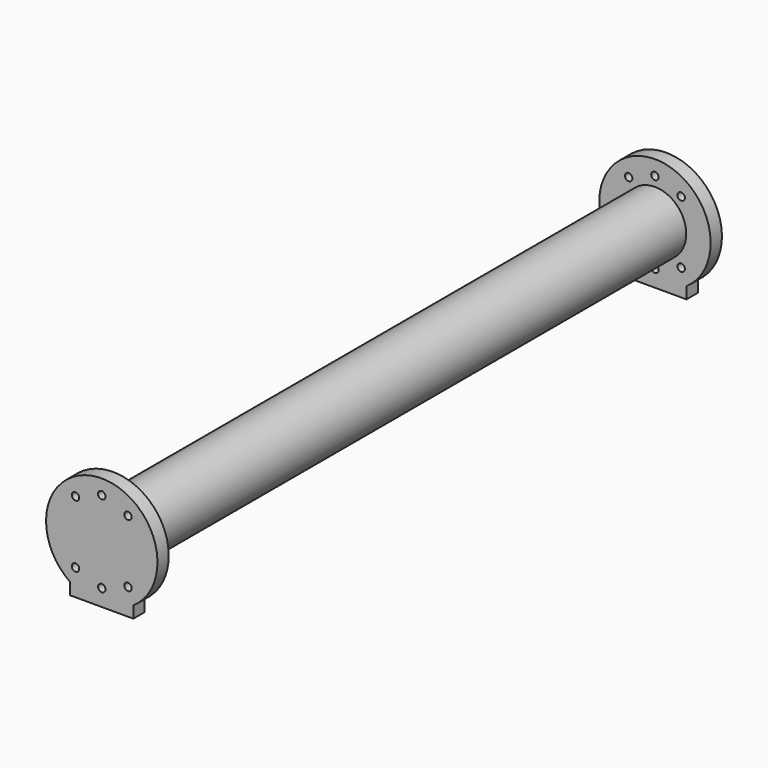
from build123d import *

# Parameters (mm, degrees)
F0_R      = 84.2
F0_R_2    = 76.2
F1_DEPTH  = 912
F2_R      = 75
F3_DEPTH  = 10
F4_R      = 10
F5_DEPTH  = 10
F8_DEPTH  = 38
F9_R      = 10
F10_DEPTH = 38


# Not quite as in the source:
# - a pattern or mirror of a feature is missing from the dataset's text; its kind, count and spacing are read off the source's solid
# - a feature names something its author has since deleted; it is built from what else it names


with BuildPart() as f1:
    # F0 (on Front) → F1 (new body, symmetric)
    with BuildSketch(Plane.XZ):
        Circle(F0_R)
        Circle(F0_R_2, mode=Mode.SUBTRACT)
    extrude(amount=F1_DEPTH, both=True)

    # F7 (on face) → F8 (join)
    with BuildSketch(Plane.XZ.offset(912)):
        with BuildLine():
            Line((85, -155), (85, -123.5920709431))
            ThreePointArc((85, -123.5920709431), (0, 150), (-85, -123.5920709431))
            Line((-85, -123.5920709431), (-85, -155))
            Line((-85, -155), (85, -155))
        make_face()
    f8 = extrude(amount=F8_DEPTH)

    # F8_copies: F8 across plane
    add(f8.mirror(Plane.ZX))

    # F9 (on face) → F10 (cut, through all)
    with BuildSketch(Plane.XZ.offset(950)):
        with Locations((-70.7066370655, 84.2648887431)):
            Circle(F9_R)
        with Locations((0, 110)):
            Circle(F9_R)
        with Locations((70.7066370655, 84.2648887431)):
            Circle(F9_R)
        with Locations((-70.7066370655, -84.2648887431)):
            Circle(F9_R)
        with Locations((0, -110)):
            Circle(F9_R)
        with Locations((70.7066370655, -84.2648887431)):
            Circle(F9_R)
    f10 = extrude(amount=-F10_DEPTH, mode=Mode.SUBTRACT)

    # F10_copies: F10 across plane
    add(f10.mirror(Plane.ZX), mode=Mode.SUBTRACT)


with BuildPart() as f3:
    # F2 (on face) → F3 (new body)
    with BuildSketch(Plane.XZ.offset(912)):
        Circle(F2_R)
    extrude(amount=F3_DEPTH)

    # F4 (on face) → F5 (cut, through all)
    with BuildSketch(Plane.XZ.offset(922)):
        with Locations((0, 61)):
            Circle(F4_R)
        with Locations((-52.8275496309, 30.5)):
            Circle(F4_R)
        with Locations((-52.8275496309, -30.5)):
            Circle(F4_R)
        with Locations((0, -61)):
            Circle(F4_R)
        with Locations((52.8275496309, -30.5)):
            Circle(F4_R)
        with Locations((52.8275496309, 30.5)):
            Circle(F4_R)
    extrude(amount=-F5_DEPTH, mode=Mode.SUBTRACT)


solid = f1.part
